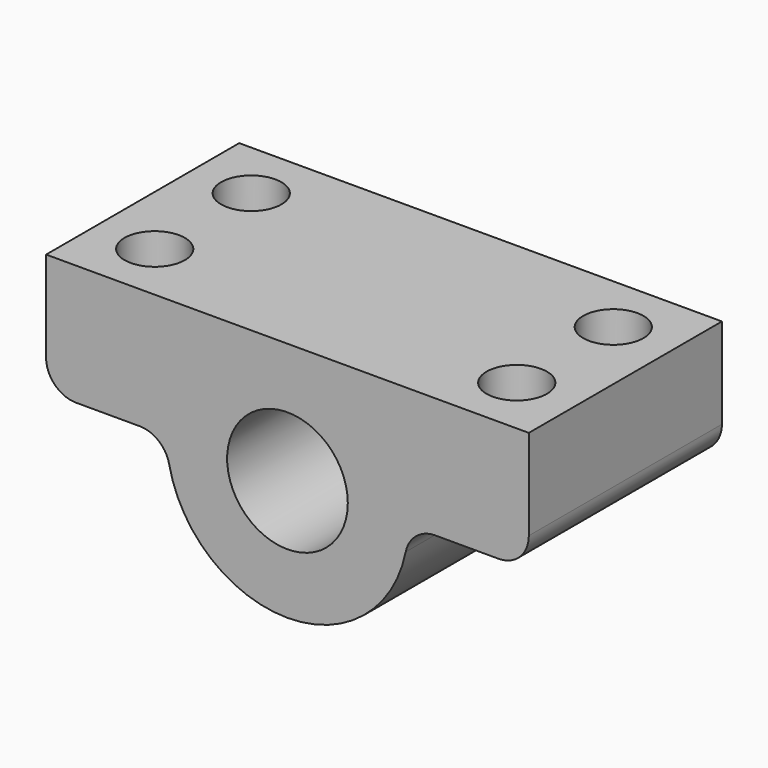
from build123d import *

# Parameters (mm, degrees)
F0_R     = 10
F1_DEPTH = 40
F3_D     = 10


# Not quite as in the source:
# - a feature names something its author has since deleted; it is built from what else it names


with BuildPart() as f1:
    # F0 (on Front) → F1 (new body)
    with BuildSketch(Plane.XZ):
        with BuildLine():
            ThreePointArc((-24.4948974278, 0), (-21.3326197677, -1.1270166538), (-19.5959179423, -4))
            ThreePointArc((-19.5959179423, -4), (0, -20), (19.5959179423, -4))
            ThreePointArc((19.5959179423, -4), (21.3326197677, -1.1270166538), (24.4948974278, 0))
            Line((24.4948974278, 0), (35, 0))
            ThreePointArc((35, 0), (38.5355339059, 1.4644660941), (40, 5))
            Line((40, 5), (40, 20))
            Line((40, 20), (-40, 20))
            Line((-40, 20), (-40, 5.3399834782))
            ThreePointArc((-40, 5.3399834782), (-38.6653317972, 1.5867843161), (-35.0115722683, 0))
            Line((-35.0115722683, 0), (-24.4948974278, 0))
        make_face()
        Circle(F0_R, mode=Mode.SUBTRACT)
    extrude(amount=F1_DEPTH)

    # F3 (through all)
    with Locations(Plane.XY.offset(20)):
        with Locations((-30, -10), (-29.9999981744, -30), (30, -30), (30, -10)):
            Hole(F3_D / 2)


solid = f1.part
